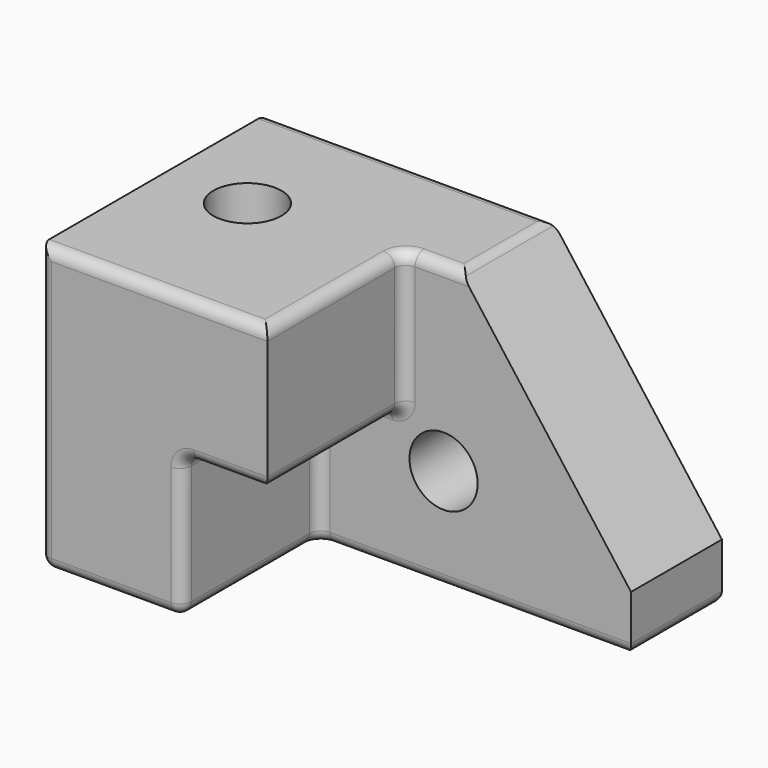
from build123d import *

# Parameters (mm, degrees)
F0_W     = 203.2
F0_H     = 127
F1_DEPTH = 127
F3_DEPTH = 76.2
F4_SIZE2 = 101.6
F4_SIZE  = 76.2
F5_R     = 5.08
F6_R     = 15.24
F7_DEPTH = 50.8
F8_R     = 15.24
F9_DEPTH = 127


with BuildPart() as f1:
    # F0 (on Front) → F1 (new body)
    with BuildSketch(Plane.XZ):
        Rectangle(F0_W, F0_H)
    extrude(amount=F1_DEPTH)

    # F2 (on face) → F3 (cut)
    with BuildSketch(Plane.XZ.offset(127)):
        Polygon((-38.1, 0), (-38.1, -63.5), (101.6, -63.5), (101.6, 63.5), (0, 63.5), (0, 0), align=None)
    extrude(amount=-F3_DEPTH, mode=Mode.SUBTRACT)

    # F4
    f4_edges = [f1.edges().sort_by_distance(p)[0] for p in [
        (101.6, -25.4, 63.5),
    ]]
    f4_side = f1.faces().sort_by_distance((-21.771429, -52.614286, 63.5))[0]
    chamfer(f4_edges, length=F4_SIZE, length2=F4_SIZE2, reference=f4_side)

    # F5
    f5_edges = [f1.edges().sort_by_distance(p)[0] for p in [
        (-50.8, -127, 63.5),
        (-19.05, -127, 0),
        (0, -88.9, 63.5),
        (0, -88.9, 0),
        (12.7, -50.8, 63.5),
        (25.4, -25.4, 63.5),
        (-38.1, 0, 63.5),
        (-38.1, -88.9, -63.5),
        (-69.85, -127, -63.5),
        (-38.1, -127, -31.75),
        (-101.6, -127, 0),
        (31.75, -50.8, -63.5),
        (101.6, -25.4, -63.5),
        (-38.1, -50.8, -31.75),
        (0, -50.8, 31.75),
        (-38.1, -88.9, 0),
        (0, 0, -63.5),
        (-101.6, -63.5, -63.5),
        (-101.6, 0, 0),
        (-19.05, -50.8, 0),
    ]]
    fillet(f5_edges, radius=F5_R)

    # F6 (on face) → F7 (cut, through all)
    with BuildSketch(Plane.XZ.offset(50.8)):
        with Locations((17.78, -17.78)):
            Circle(F6_R)
    extrude(amount=-F7_DEPTH, mode=Mode.SUBTRACT)

    # F8 (on face) → F9 (cut, through all)
    with BuildSketch(Plane.XY.offset(63.5)):
        with Locations((-64.6355301142, -57.3951564729)):
            Circle(F8_R)
    extrude(amount=-F9_DEPTH, mode=Mode.SUBTRACT)


solid = f1.part
